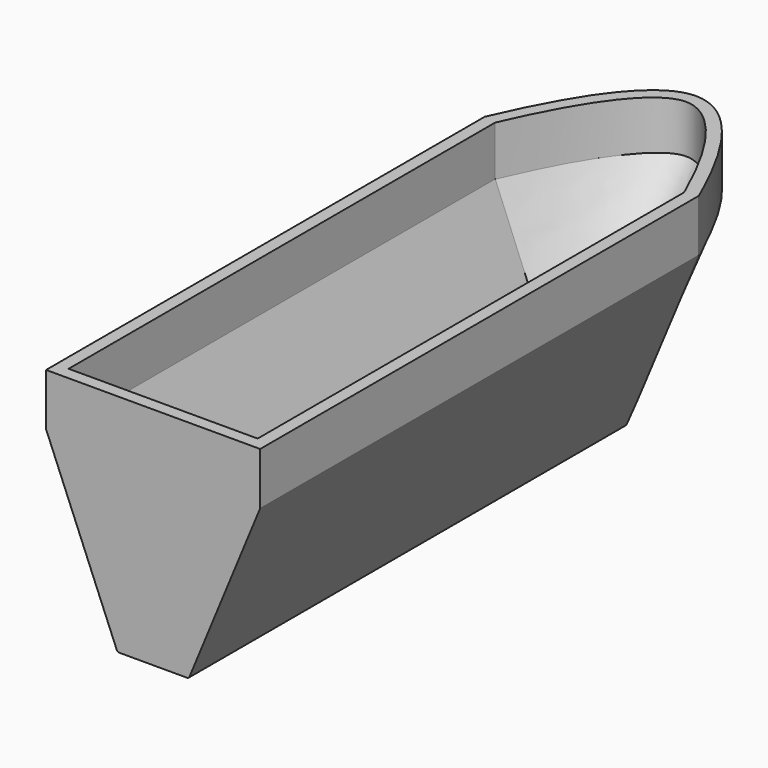
from build123d import *

# Parameters (mm, degrees)
F2_W     = 13.66667
F2_H     = 105
F4_DEPTH = 10
F5_T     = -2.4
F6_R     = 0.5


with BuildPart() as f3:
    # F1 (on offset) → F3 section 0
    with BuildSketch(Plane.XY.offset(33.125)):
        with BuildLine():
            add(Edge.make_bspline(
                [(-20.5, 0), (-14, 15), (0, 35), (14, 15), (20.5, 0)],
                knots=[0, 0, 0, 0, 0.5, 1, 1, 1, 1], degree=3))
            Line((-20.5, 0), (-20.5, -105))
            Line((-20.5, -105), (20.5, -105))
            Line((20.5, -105), (20.5, 0))
        make_face()
    # F2 (on Top) → F3 section 1
    with BuildSketch(Plane.XY):
        with Locations((-3.5e-05, -52.5)):
            Rectangle(F2_W, F2_H)
    loft()

    # F4 (add): a face of the model
    f4_faces = [f3.faces().sort_by_distance(p)[0] for p in [
        (4.4104e-06, -44.0610349969, 33.125),
    ]]
    extrude(f4_faces, amount=F4_DEPTH)

    # F5
    f5_openings = [f3.faces().sort_by_distance(p)[0] for p in [
        (4e-06, -44.061035, 43.125),
    ]]
    offset(amount=F5_T, openings=f5_openings)

    # F6
    f6_edges = [f3.edges().sort_by_distance(p)[0] for p in [
        (-6.83337, -52.5, 0),
        (6.8333, -52.5, 0),
        (-3.5e-05, 0, 0),
        (13.66665, 0, 16.5625),
        (-13.666685, 0, 16.5625),
    ]]
    fillet(f6_edges, radius=F6_R)


solid = f3.part
